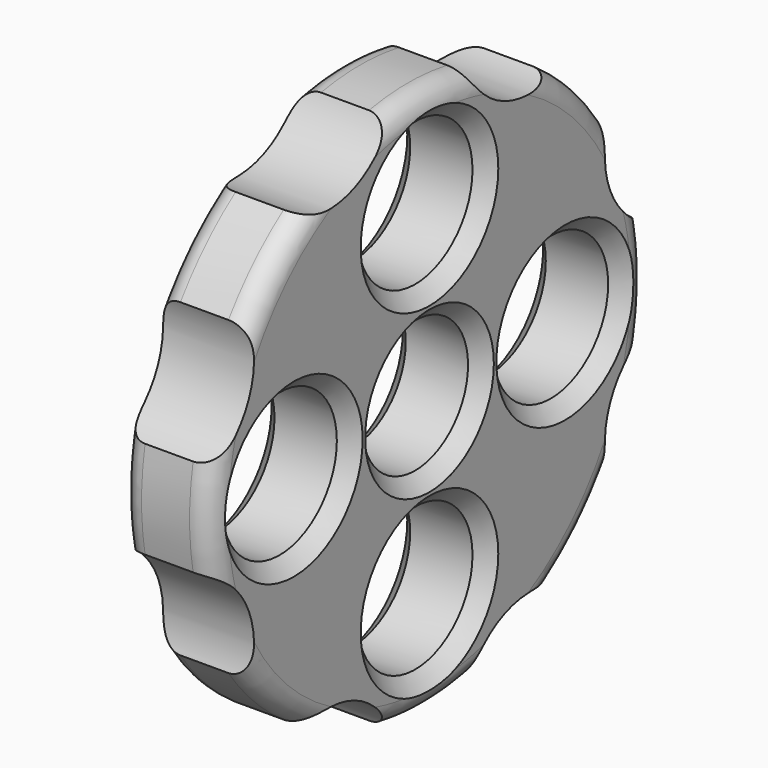
from build123d import *

# Parameters (mm, degrees)
F0_R     = 19.05
F0_R_2   = 4.6125
F1_DEPTH = 6.35
F2_R     = 5
F3_DEPTH = 6.351
F4_SIZE  = 1
F6_R     = 5.9511153658
F7_DEPTH = 6.3510001


# Not quite as in the source:
# - a fillet or chamfer that OpenCascade refuses, or shapes differently, is made with other operations: its cross-section is extruded or revolved along the edge and cut away or added


with BuildPart() as f1:
    # F0 (on Right) → F1 (new body)
    with BuildSketch(Plane.YZ):
        Circle(F0_R)
        Circle(F0_R_2, mode=Mode.SUBTRACT)
    extrude(amount=F1_DEPTH)

    # F2 (on face) → F3 (cut, through all)
    with BuildSketch(Plane.YZ.offset(6.35)):
        with Locations((0, 11.83125)):
            Circle(F2_R)
        with Locations((-11.83125, 0)):
            Circle(F2_R)
        with Locations((0, -11.83125)):
            Circle(F2_R)
        with Locations((11.83125, 0)):
            Circle(F2_R)
    extrude(amount=-F3_DEPTH, mode=Mode.SUBTRACT)

    # F4
    f4_edges = [f1.edges().sort_by_distance(p)[0] for p in [
        (6.35, -5, 11.83125),
        (0, -5, 11.83125),
        (6.35, -4.6125, 0),
        (0, -4.6125, 0),
        (6.35, 6.83125, 0),
        (0, 6.83125, 0),
        (0, -16.83125, 0),
        (6.35, -16.83125, 0),
        (0, -5, -11.83125),
        (6.35, -5, -11.83125),
    ]]
    chamfer(f4_edges, length=F4_SIZE)

    # F5: fillet of radius 1.5 on 2 edges, made by hand

    # F5_s1 → F5_t2 (revolve, cut)
    with BuildSketch(Plane.XY):
        with BuildLine():
            ThreePointArc((4.85, 19.05), (5.9106601718, 18.6106601718), (6.35, 17.55))
            Line((6.35, 17.55), (6.35, 19.05))
            Line((6.35, 19.05), (4.85, 19.05))
        make_face()
    revolve(axis=Axis((6.35, 0, 0), (1, 0, 0)), mode=Mode.SUBTRACT)

    # F5_s3 → F5_t4 (revolve, cut)
    with BuildSketch(Plane.XY):
        with BuildLine():
            ThreePointArc((0, 17.55), (0.4393398282, 18.6106601718), (1.5, 19.05))
            Line((1.5, 19.05), (0, 19.05))
            Line((0, 19.05), (0, 17.55))
        make_face()
    revolve(axis=Axis((0, 0, 0), (1, 0, 0)), mode=Mode.SUBTRACT)

    # F6 (on face) → F7 (cut, through all)
    with BuildSketch(Plane.YZ.offset(6.35)):
        with Locations((8.8021457764, 21.2502597114)):
            Circle(F6_R)
        with Locations((-8.8021457764, 21.2502597114)):
            Circle(F6_R)
        with Locations((-21.2502597114, 8.8021457764)):
            Circle(F6_R)
        with Locations((-21.2502597114, -8.8021457764)):
            Circle(F6_R)
        with Locations((-8.8021457764, -21.2502597114)):
            Circle(F6_R)
        with Locations((8.8021457764, -21.2502597114)):
            Circle(F6_R)
        with Locations((21.2502597114, -8.8021457764)):
            Circle(F6_R)
        with Locations((21.2502597114, 8.8021457764)):
            Circle(F6_R)
    extrude(amount=-F7_DEPTH, mode=Mode.SUBTRACT)


solid = f1.part
